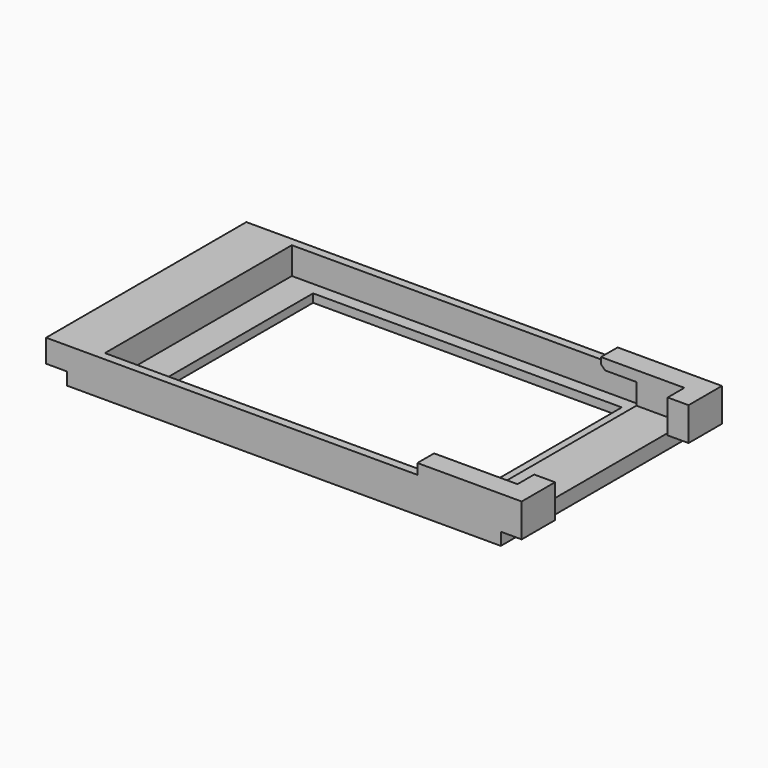
from build123d import *

# Parameters (mm, degrees)
F0_W      = 104
F0_H      = 60
F0_W_2    = 85
F0_H_2    = 56
F1_DEPTH  = 8.5
F2_DEPTH  = 2
F3_W      = 8.5
F3_H      = 3
F4_DEPTH  = 2.5
F5_SIZE   = 1
F6_DEPTH  = 5
F7_W      = 5
F7_H      = 10
F8_DEPTH  = 8
F9_W      = 5
F9_H      = 60
F10_DEPTH = 5.5


with BuildPart() as f1:
    # F0 (on Top) → F1 (new body)
    with BuildSketch(Plane.XY):
        with Locations((1.1924776137, -7.5798341542)):
            Rectangle(F0_W, F0_H)
        with Locations((-0.8075223863, -7.5798341542)):
            Rectangle(F0_W_2, F0_H_2, mode=Mode.SUBTRACT)
    extrude(amount=F1_DEPTH)

    # F0 (on Top) → F2 (join)
    with BuildSketch(Plane.XY):
        with Locations((-0.8075223863, -7.5798341542)):
            Rectangle(F0_W_2, F0_H_2)
        Polygon((-35.8075223863, -32.5798341542), (-35.8075223863, 17.4201658458), (34.1924776137, 17.4201658458), (38.1924776137, 17.4201658458), (38.1924776137, -32.5798341542), align=None, mode=Mode.SUBTRACT)
    extrude(amount=F2_DEPTH)

    # F3 (on face) → F4 (join)
    with BuildSketch(Plane.XY.offset(8.5)):
        with Locations((37.4424776137, -34.0798341542)):
            Rectangle(F3_W, F3_H)
        with Locations((37.4424776137, 18.9201658458)):
            Rectangle(F3_W, F3_H)
        Polygon((33.1924776137, -37.5798341542), (53.1924776137, -37.5798341542), (53.1924776137, -32.5798341542), (41.6924776137, -32.5798341542), (41.6924776137, -35.5798341542), (33.1924776137, -35.5798341542), align=None)
        Polygon((41.6924776137, 17.4201658458), (53.1924776137, 17.4201658458), (53.1924776137, 22.4201658458), (33.1924776137, 22.4201658458), (33.1924776137, 20.4201658458), (41.6924776137, 20.4201658458), align=None)
    extrude(amount=F4_DEPTH)

    # F5
    f5_edges = [f1.edges().sort_by_distance(p)[0] for p in [
        (33.192478, 18.920166, 8.5),
        (33.192478, -34.079834, 8.5),
    ]]
    chamfer(f5_edges, length=F5_SIZE)

    # F6 (cut): a face of the model
    f6_faces = [f1.faces().sort_by_distance(p)[0] for p in [
        (47.4424776137, -7.5798341542, 8.5),
    ]]
    extrude(f6_faces, amount=-F6_DEPTH, mode=Mode.SUBTRACT)

    # F7 (on face) → F8 (join)
    with BuildSketch(Plane.XY.offset(11)):
        Polygon((53.1924776137, 17.4201658458), (53.1924776137, 12.4201658458), (58.1924776137, 12.4201658458), (58.1924776137, 22.4201658458), (53.1924776137, 22.4201658458), align=None)
        with Locations((55.6924776137, -32.5798341542)):
            Rectangle(F7_W, F7_H)
    extrude(amount=-F8_DEPTH)

    # F9 (on face) → F10 (join)
    with BuildSketch(Plane.XY.offset(8.5)):
        with Locations((-53.3075223863, -7.5798341542)):
            Rectangle(F9_W, F9_H)
    extrude(amount=-F10_DEPTH)


solid = f1.part
